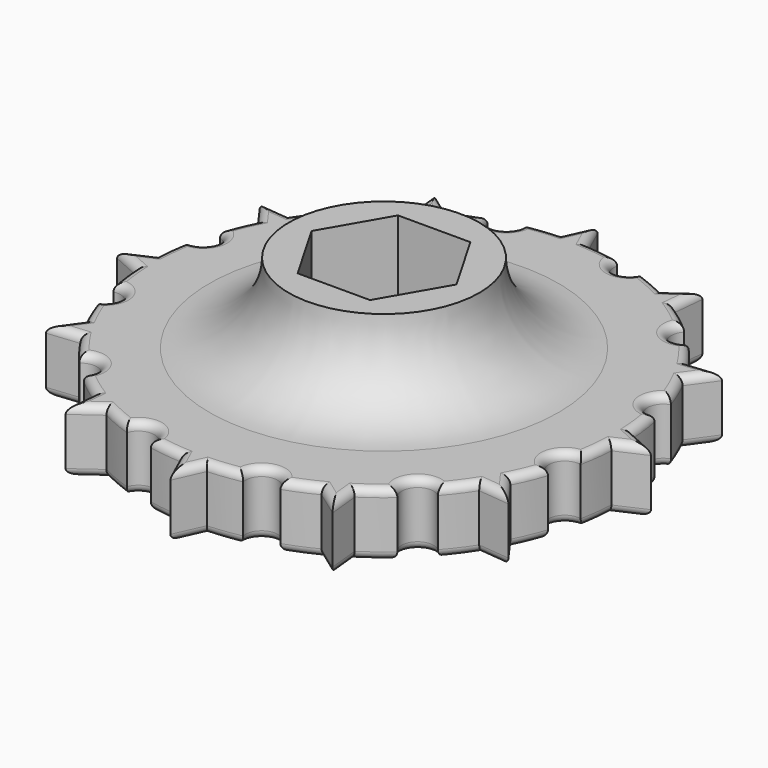
from build123d import *

# Parameters (mm, degrees)
F1_DEPTH = 4
F2_R     = 6
F3_DEPTH = 5
F4_R     = 4.99999
F5_R     = 0.5


# Not quite as in the source:
# - a fillet or chamfer is up to 0.001 mm smaller than in the source, because OpenCascade refuses the exact size


with BuildPart() as f1:
    # F0 (on Top) → F1 (new body)
    with BuildSketch(Plane.XY):
        with BuildLine():
            Line((0, 16.8088469654), (-0.8241778737, 14.9773405794))
            ThreePointArc((-0.8241778737, 14.9773405794), (-1.8708148785, 14.8828778027), (-2.9082693233, 14.7153650836))
            ThreePointArc((-2.9082693233, 14.7153650836), (-3.6234666314, 13.522961568), (-4.8390474267, 14.19801465))
            ThreePointArc((-4.8390474267, 14.19801465), (-5.8212656908, 13.8243576978), (-6.7749113139, 13.3828463598))
            Line((-6.7749113139, 13.3828463598), (-8.4044234827, 14.5568884804))
            Line((-8.4044234827, 14.5568884804), (-8.2024292656, 12.5586684861))
            ThreePointArc((-8.2024292656, 12.5586684861), (-9.061612112, 11.9535428193), (-9.8763176569, 11.2897453267))
            ThreePointArc((-9.8763176569, 11.2897453267), (-9.8994949366, 9.8994949366), (-11.2897453267, 9.8763176569))
            ThreePointArc((-11.2897453267, 9.8763176569), (-11.9535428193, 9.061612112), (-12.5586684861, 8.2024292656))
            Line((-12.5586684861, 8.2024292656), (-14.5568884804, 8.4044234827))
            Line((-14.5568884804, 8.4044234827), (-13.3828463598, 6.7749113139))
            ThreePointArc((-13.3828463598, 6.7749113139), (-13.8243576978, 5.8212656908), (-14.19801465, 4.8390474267))
            ThreePointArc((-14.19801465, 4.8390474267), (-13.522961568, 3.6234666314), (-14.7153650836, 2.9082693233))
            ThreePointArc((-14.7153650836, 2.9082693233), (-14.8828778027, 1.8708148785), (-14.9773405794, 0.8241778737))
            Line((-14.9773405794, 0.8241778737), (-16.8088469654, 0))
            Line((-16.8088469654, 0), (-14.9773405794, -0.8241778737))
            ThreePointArc((-14.9773405794, -0.8241778737), (-14.8828778027, -1.8708148785), (-14.7153650836, -2.9082693233))
            ThreePointArc((-14.7153650836, -2.9082693233), (-13.522961568, -3.6234666314), (-14.19801465, -4.8390474267))
            ThreePointArc((-14.19801465, -4.8390474267), (-13.8243576978, -5.8212656908), (-13.3828463598, -6.7749113139))
            Line((-13.3828463598, -6.7749113139), (-14.5568884804, -8.4044234827))
            Line((-14.5568884804, -8.4044234827), (-12.5586684861, -8.2024292656))
            ThreePointArc((-12.5586684861, -8.2024292656), (-11.9535428193, -9.061612112), (-11.2897453267, -9.8763176569))
            ThreePointArc((-11.2897453267, -9.8763176569), (-9.8994949366, -9.8994949366), (-9.8763176569, -11.2897453267))
            ThreePointArc((-9.8763176569, -11.2897453267), (-9.061612112, -11.9535428193), (-8.2024292656, -12.5586684861))
            Line((-8.2024292656, -12.5586684861), (-8.4044234827, -14.5568884804))
            Line((-8.4044234827, -14.5568884804), (-6.7749113139, -13.3828463598))
            ThreePointArc((-6.7749113139, -13.3828463598), (-5.8212656908, -13.8243576978), (-4.8390474267, -14.19801465))
            ThreePointArc((-4.8390474267, -14.19801465), (-3.6234666314, -13.522961568), (-2.9082693233, -14.7153650836))
            ThreePointArc((-2.9082693233, -14.7153650836), (-1.8708148785, -14.8828778027), (-0.8241778737, -14.9773405794))
            Line((-0.8241778737, -14.9773405794), (0, -16.8088469654))
            Line((0, -16.8088469654), (0.8241778737, -14.9773405794))
            ThreePointArc((0.8241778737, -14.9773405794), (1.8708148785, -14.8828778027), (2.9082693233, -14.7153650836))
            ThreePointArc((2.9082693233, -14.7153650836), (3.6234666314, -13.522961568), (4.8390474267, -14.19801465))
            ThreePointArc((4.8390474267, -14.19801465), (5.8212656908, -13.8243576978), (6.7749113139, -13.3828463598))
            Line((6.7749113139, -13.3828463598), (8.4044234827, -14.5568884804))
            Line((8.4044234827, -14.5568884804), (8.2024292656, -12.5586684861))
            ThreePointArc((8.2024292656, -12.5586684861), (9.061612112, -11.9535428193), (9.8763176569, -11.2897453267))
            ThreePointArc((9.8763176569, -11.2897453267), (9.8994949366, -9.8994949366), (11.2897453267, -9.8763176569))
            ThreePointArc((11.2897453267, -9.8763176569), (11.9535428193, -9.061612112), (12.5586684861, -8.2024292656))
            Line((12.5586684861, -8.2024292656), (14.5568884804, -8.4044234827))
            Line((14.5568884804, -8.4044234827), (13.3828463598, -6.7749113139))
            ThreePointArc((13.3828463598, -6.7749113139), (13.8243576978, -5.8212656908), (14.19801465, -4.8390474267))
            ThreePointArc((14.19801465, -4.8390474267), (13.522961568, -3.6234666314), (14.7153650836, -2.9082693233))
            ThreePointArc((14.7153650836, -2.9082693233), (14.8828778027, -1.8708148785), (14.9773405794, -0.8241778737))
            Line((14.9773405794, -0.8241778737), (16.8088469654, 0))
            Line((16.8088469654, 0), (14.9773405794, 0.8241778737))
            ThreePointArc((14.9773405794, 0.8241778737), (14.8828778027, 1.8708148785), (14.7153650836, 2.9082693233))
            ThreePointArc((14.7153650836, 2.9082693233), (13.522961568, 3.6234666314), (14.19801465, 4.8390474267))
            ThreePointArc((14.19801465, 4.8390474267), (13.8243576978, 5.8212656908), (13.3828463598, 6.7749113139))
            Line((13.3828463598, 6.7749113139), (14.5568884804, 8.4044234827))
            Line((14.5568884804, 8.4044234827), (12.5586684861, 8.2024292656))
            ThreePointArc((12.5586684861, 8.2024292656), (11.9535428193, 9.061612112), (11.2897453267, 9.8763176569))
            ThreePointArc((11.2897453267, 9.8763176569), (9.8994949366, 9.8994949366), (9.8763176569, 11.2897453267))
            ThreePointArc((9.8763176569, 11.2897453267), (9.061612112, 11.9535428193), (8.2024292656, 12.5586684861))
            Line((8.2024292656, 12.5586684861), (8.4044234827, 14.5568884804))
            Line((8.4044234827, 14.5568884804), (6.7749113139, 13.3828463598))
            ThreePointArc((6.7749113139, 13.3828463598), (5.8212656908, 13.8243576978), (4.8390474267, 14.19801465))
            ThreePointArc((4.8390474267, 14.19801465), (3.6234666314, 13.522961568), (2.9082693233, 14.7153650836))
            ThreePointArc((2.9082693233, 14.7153650836), (1.8708148785, 14.8828778027), (0.8241778737, 14.9773405794))
            Line((0.8241778737, 14.9773405794), (0, 16.8088469654))
        make_face()
        with BuildLine():
            ThreePointArc((-2.5, 0), (-1.767766953, 1.767766953), (0, 2.5))
            ThreePointArc((0, 2.5), (1.767766953, 1.767766953), (2.5, 0))
            ThreePointArc((2.5, 0), (1.767766953, -1.767766953), (0, -2.5))
            ThreePointArc((0, -2.5), (-1.767766953, -1.767766953), (-2.5, 0))
        make_face(mode=Mode.SUBTRACT)
    extrude(amount=F1_DEPTH)

    # F2 (on face) → F3 (join)
    with BuildSketch(Plane.XY.offset(4)):
        Circle(F2_R)
        Polygon((-4.5610671266, 0), (-2.2805335633, 3.95), (2.2805335633, 3.95), (4.5610671266, 0), (2.2805335633, -3.95), (-2.2805335633, -3.95), align=None, mode=Mode.SUBTRACT)
    extrude(amount=F3_DEPTH)

    # F4 (radius 5 in the source; OpenCascade refuses exactly that, so slightly less here)
    f4_edges = [f1.edges().sort_by_distance(p)[0] for p in [
        (-6, 0, 4),
    ]]
    fillet(f4_edges, radius=F4_R)

    # F5
    f5_edges = [f1.edges().sort_by_distance(p)[0] for p in [
        (-10.99999, 0, 4),
        (0.412089, 15.893094, 4),
        (1.870815, 14.882878, 4),
        (-0.412089, 15.893094, 4),
        (3.623467, 13.522962, 4),
        (-1.870815, 14.882878, 4),
        (5.821266, 13.824358, 4),
        (-3.623467, 13.522962, 4),
        (7.589667, 13.969867, 4),
        (-5.821266, 13.824358, 4),
        (8.303426, 13.557778, 4),
        (-7.589667, 13.969867, 4),
        (9.061612, 11.953543, 4),
        (-8.303426, 13.557778, 4),
        (9.899495, 9.899495, 4),
        (-9.061612, 11.953543, 4),
        (11.953543, 9.061612, 4),
        (-9.899495, 9.899495, 4),
        (13.557778, 8.303426, 4),
        (-11.953543, 9.061612, 4),
        (13.969867, 7.589667, 4),
        (-13.557778, 8.303426, 4),
        (13.824358, 5.821266, 4),
        (-13.969867, 7.589667, 4),
        (13.522962, 3.623467, 4),
        (-13.824358, 5.821266, 4),
        (14.882878, 1.870815, 4),
        (-13.522962, 3.623467, 4),
        (15.893094, 0.412089, 4),
        (-14.882878, 1.870815, 4),
        (15.893094, -0.412089, 4),
        (-15.893094, 0.412089, 4),
        (14.882878, -1.870815, 4),
        (-15.893094, -0.412089, 4),
        (13.522962, -3.623467, 4),
        (-14.882878, -1.870815, 4),
        (13.824358, -5.821266, 4),
        (-13.522962, -3.623467, 4),
        (13.969867, -7.589667, 4),
        (-13.824358, -5.821266, 4),
        (13.557778, -8.303426, 4),
        (-13.969867, -7.589667, 4),
        (11.953543, -9.061612, 4),
        (-13.557778, -8.303426, 4),
        (9.899495, -9.899495, 4),
        (-11.953543, -9.061612, 4),
        (9.061612, -11.953543, 4),
        (-9.899495, -9.899495, 4),
        (8.303426, -13.557778, 4),
        (-9.061612, -11.953543, 4),
        (7.589667, -13.969867, 4),
        (-8.303426, -13.557778, 4),
        (5.821266, -13.824358, 4),
        (-7.589667, -13.969867, 4),
        (3.623467, -13.522962, 4),
        (-5.821266, -13.824358, 4),
        (1.870815, -14.882878, 4),
        (-3.623467, -13.522962, 4),
        (0.412089, -15.893094, 4),
        (-1.870815, -14.882878, 4),
        (-0.412089, -15.893094, 4),
        (0.412089, 15.893094, 0),
        (-0.412089, 15.893094, 0),
        (-1.870815, 14.882878, 0),
        (-3.623467, 13.522962, 0),
        (-5.821266, 13.824358, 0),
        (-7.589667, 13.969867, 0),
        (-8.303426, 13.557778, 0),
        (-9.061612, 11.953543, 0),
        (-9.899495, 9.899495, 0),
        (-11.953543, 9.061612, 0),
        (-13.557778, 8.303426, 0),
        (-13.969867, 7.589667, 0),
        (-13.824358, 5.821266, 0),
        (-13.522962, 3.623467, 0),
        (-14.882878, 1.870815, 0),
        (-15.893094, 0.412089, 0),
        (-15.893094, -0.412089, 0),
        (-14.882878, -1.870815, 0),
        (-13.522962, -3.623467, 0),
        (-13.824358, -5.821266, 0),
        (-13.969867, -7.589667, 0),
        (-13.557778, -8.303426, 0),
        (-11.953543, -9.061612, 0),
        (-9.899495, -9.899495, 0),
        (-9.061612, -11.953543, 0),
        (-8.303426, -13.557778, 0),
        (-7.589667, -13.969867, 0),
        (-5.821266, -13.824358, 0),
        (-3.623467, -13.522962, 0),
        (-1.870815, -14.882878, 0),
        (-0.412089, -15.893094, 0),
        (0.412089, -15.893094, 0),
        (1.870815, -14.882878, 0),
        (3.623467, -13.522962, 0),
        (5.821266, -13.824358, 0),
        (7.589667, -13.969867, 0),
        (8.303426, -13.557778, 0),
        (9.061612, -11.953543, 0),
        (9.899495, -9.899495, 0),
        (11.953543, -9.061612, 0),
        (13.557778, -8.303426, 0),
        (13.969867, -7.589667, 0),
        (13.824358, -5.821266, 0),
        (13.522962, -3.623467, 0),
        (14.882878, -1.870815, 0),
        (15.893094, -0.412089, 0),
        (15.893094, 0.412089, 0),
        (14.882878, 1.870815, 0),
        (13.522962, 3.623467, 0),
        (13.824358, 5.821266, 0),
        (13.969867, 7.589667, 0),
        (13.557778, 8.303426, 0),
        (11.953543, 9.061612, 0),
        (9.899495, 9.899495, 0),
        (9.061612, 11.953543, 0),
        (8.303426, 13.557778, 0),
        (7.589667, 13.969867, 0),
        (5.821266, 13.824358, 0),
        (3.623467, 13.522962, 0),
        (1.870815, 14.882878, 0),
        (2.5, 0, 0),
    ]]
    fillet(f5_edges, radius=F5_R)


solid = f1.part
